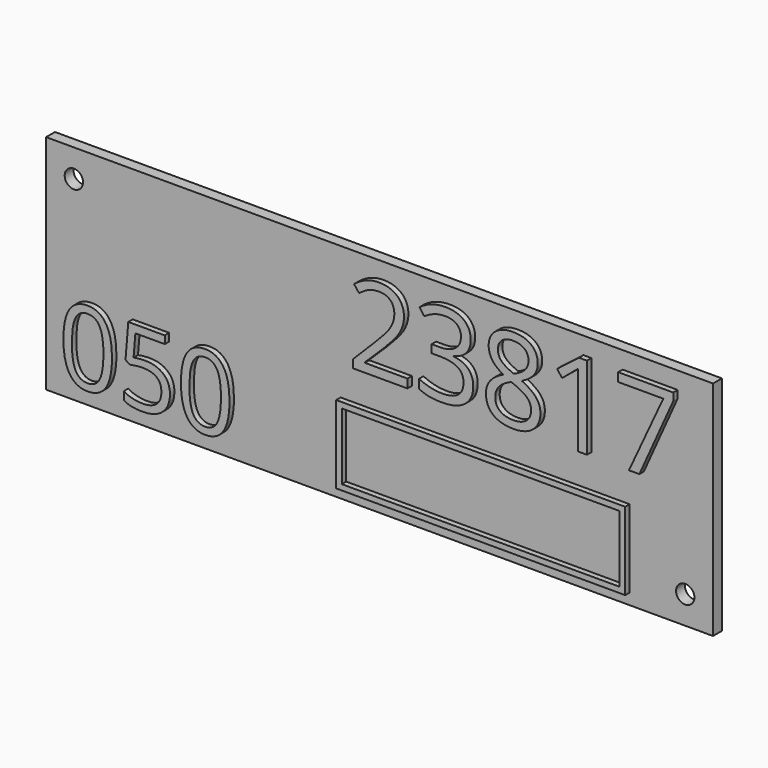
from build123d import *

# Parameters (mm, degrees)
F0_W         = 120
F0_H         = 40
F1_DEPTH     = 2
F3_D         = 3.3
F4_TEXT_SIZE = 20.8865923307
F5_DEPTH     = 1
F6_TEXT_SIZE = 18.4937691891
F7_DEPTH     = 1
F8_W         = 52
F8_H         = 14
F8_W_2       = 49.99999962
F8_H_2       = 11.99999962
F9_DEPTH     = 1


# Not quite as in the source:
# - Text() gives the source's letters only with a copy of the font that has no kerning and outlines rounded to 1/6400 em; it was checked with that copy


with BuildPart() as f1:
    # F0 (on Front) → F1 (new body)
    with BuildSketch(Plane.XZ):
        Rectangle(F0_W, F0_H)
    extrude(amount=F1_DEPTH)

    # F3 (through all)
    with Locations(Plane.XZ.offset(2)):
        with Locations((-55, 15), (55, -15)):
            Hole(F3_D / 2)

    # F4 (on face) → F5 (join)
    with BuildSketch(Plane.XZ.offset(2)):
        with Locations((-5, 2)):
            Text('23817', F4_TEXT_SIZE, font='Open Sans', text_align=(TextAlign.LEFT, TextAlign.BOTTOM))
    extrude(amount=F5_DEPTH)

    # F6 (on face) → F7 (join)
    with BuildSketch(Plane.XZ.offset(2)):
        with Locations((-57, -17)):
            Text('050', F6_TEXT_SIZE, font='Open Sans', text_align=(TextAlign.LEFT, TextAlign.BOTTOM))
    extrude(amount=F7_DEPTH)

    # F8 (on face) → F9 (join)
    with BuildSketch(Plane.XZ.offset(2)):
        with Locations((19, -11)):
            Rectangle(F8_W, F8_H)
        with Locations((19, -11)):
            Rectangle(F8_W_2, F8_H_2, mode=Mode.SUBTRACT)
    extrude(amount=F9_DEPTH)


solid = f1.part
